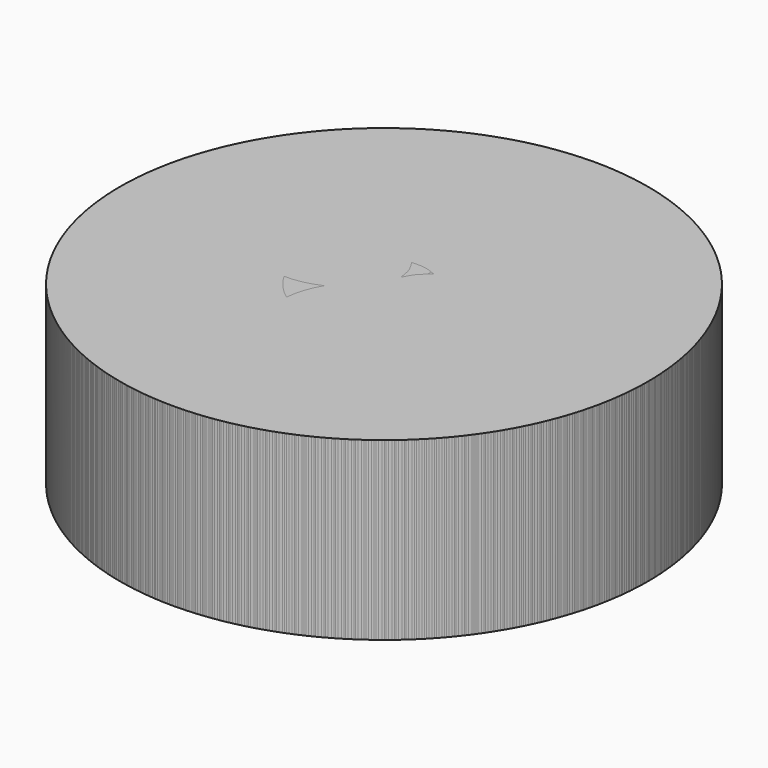
from build123d import *

# Parameters (mm, degrees)
F1_R      = 90
F2_DEPTH  = 60
F3_R      = 85
F3_R_2    = 75
F4_DEPTH  = 4
F5_R      = 75
F7_DEPTH  = 50
F8_DEPTH  = 10
F9_COUNT  = 9
F11_DEPTH = 10
F12_COUNT = 12


with BuildPart() as f2:
    # F1 (on Top) → F2 (new body)
    with BuildSketch(Plane.XY):
        Circle(F1_R)
    extrude(amount=-F2_DEPTH)

    # F3 (on face) → F4 (cut)
    with BuildSketch(Plane(origin=(0, 0, -60), x_dir=(1, 0, 0), z_dir=(0, 0, -1))):
        Circle(F3_R)
        Circle(F3_R_2, mode=Mode.SUBTRACT)
    extrude(amount=-F4_DEPTH, mode=Mode.SUBTRACT)

    # F5 (on face) → F7 (cut)
    with BuildSketch(Plane(origin=(0, 0, -60), x_dir=(1, 0, 0), z_dir=(0, 0, -1))):
        Circle(F5_R)
    extrude(amount=-F7_DEPTH, mode=Mode.SUBTRACT)

    # F0 (on Top) → F8 (cut, through all)
    with BuildSketch(Plane.XY):
        with BuildLine():
            add(Edge.make_bspline(
                [(-4.5, -13.7942286341), (-1.4705771366, -10.347114317), (-1.4705771366, -10.347114317), (0, -6)],
                knots=[0, 0, 0, 0, 9, 9, 9, 9], degree=3))
            add(Edge.make_bspline(
                [(-4.5, -13.7942286341), (0, -14.6942286341), (0, -14.6942286341), (4.5, -13.7942286341)],
                knots=[0, 0, 0, 0, 9, 9, 9, 9], degree=3))
            add(Edge.make_bspline(
                [(0, -6), (1.4705771366, -10.347114317), (1.4705771366, -10.347114317), (4.5, -13.7942286341)],
                knots=[0, 0, 0, 0, 9, 9, 9, 9], degree=3))
        make_face()
    extrude(amount=-F8_DEPTH, mode=Mode.SUBTRACT)


with BuildPart() as f9_1:
    # F9: instance of F2
    add(f2.part.rotate(Axis((0, 0, -60), (0, 0, -1)), 1 * 360 / F9_COUNT))


with BuildPart() as f9_2:
    # F9: instance of F2
    add(f2.part.rotate(Axis((0, 0, -60), (0, 0, -1)), 2 * 360 / F9_COUNT))


with BuildPart() as f9_3:
    # F9: instance of F2
    add(f2.part.rotate(Axis((0, 0, -60), (0, 0, -1)), 3 * 360 / F9_COUNT))


with BuildPart() as f9_4:
    # F9: instance of F2
    add(f2.part.rotate(Axis((0, 0, -60), (0, 0, -1)), 4 * 360 / F9_COUNT))


with BuildPart() as f9_5:
    # F9: instance of F2
    add(f2.part.rotate(Axis((0, 0, -60), (0, 0, -1)), 5 * 360 / F9_COUNT))


with BuildPart() as f9_6:
    # F9: instance of F2
    add(f2.part.rotate(Axis((0, 0, -60), (0, 0, -1)), 6 * 360 / F9_COUNT))


with BuildPart() as f9_7:
    # F9: instance of F2
    add(f2.part.rotate(Axis((0, 0, -60), (0, 0, -1)), 7 * 360 / F9_COUNT))


with BuildPart() as f9_8:
    # F9: instance of F2
    add(f2.part.rotate(Axis((0, 0, -60), (0, 0, -1)), 8 * 360 / F9_COUNT))


with BuildPart() as f11_tool:
    # F10 (on face) → F11 (new body, through all)
    with BuildSketch(Plane.XY):
        with BuildLine():
            ThreePointArc((-4.9412984546, -15.1469779182), (-8.9537537737, -19.6587371709), (-13.868495, -23.1660278519))
            ThreePointArc((-13.868495, -23.1660278519), (-8.3737215587, -25.6686732664), (-2.4601957705, -26.887681878))
            ThreePointArc((-2.4601957705, -26.887681878), (-4.3612662396, -21.1569140137), (-4.9412984546, -15.1469779182))
        make_face()
    extrude(amount=-F11_DEPTH)


with BuildPart() as f2_1:
    add(f2.part)

    # F11: cut by f11_tool
    add(f11_tool.part, mode=Mode.SUBTRACT)


with BuildPart() as f9_1_1:
    add(f9_1.part)

    # F11: cut by f11_tool
    add(f11_tool.part, mode=Mode.SUBTRACT)


with BuildPart() as f9_2_1:
    add(f9_2.part)

    # F11: cut by f11_tool
    add(f11_tool.part, mode=Mode.SUBTRACT)


with BuildPart() as f9_3_1:
    add(f9_3.part)

    # F11: cut by f11_tool
    add(f11_tool.part, mode=Mode.SUBTRACT)


with BuildPart() as f9_4_1:
    add(f9_4.part)

    # F11: cut by f11_tool
    add(f11_tool.part, mode=Mode.SUBTRACT)


with BuildPart() as f9_5_1:
    add(f9_5.part)

    # F11: cut by f11_tool
    add(f11_tool.part, mode=Mode.SUBTRACT)


with BuildPart() as f9_6_1:
    add(f9_6.part)

    # F11: cut by f11_tool
    add(f11_tool.part, mode=Mode.SUBTRACT)


with BuildPart() as f9_7_1:
    add(f9_7.part)

    # F11: cut by f11_tool
    add(f11_tool.part, mode=Mode.SUBTRACT)


with BuildPart() as f9_8_1:
    add(f9_8.part)

    # F11: cut by f11_tool
    add(f11_tool.part, mode=Mode.SUBTRACT)


with BuildPart() as f12_1:
    # F12: instance of F9_4
    add(f9_4_1.part.rotate(Axis((0, 0, 0), (0, 0, 1)), 1 * 360 / F12_COUNT))


with BuildPart() as f12_2:
    # F12: instance of F9_4
    add(f9_4_1.part.rotate(Axis((0, 0, 0), (0, 0, 1)), 2 * 360 / F12_COUNT))


with BuildPart() as f12_3:
    # F12: instance of F9_4
    add(f9_4_1.part.rotate(Axis((0, 0, 0), (0, 0, 1)), 3 * 360 / F12_COUNT))


with BuildPart() as f12_4:
    # F12: instance of F9_4
    add(f9_4_1.part.rotate(Axis((0, 0, 0), (0, 0, 1)), 4 * 360 / F12_COUNT))


with BuildPart() as f12_5:
    # F12: instance of F9_4
    add(f9_4_1.part.rotate(Axis((0, 0, 0), (0, 0, 1)), 5 * 360 / F12_COUNT))


with BuildPart() as f12_6:
    # F12: instance of F9_4
    add(f9_4_1.part.rotate(Axis((0, 0, 0), (0, 0, 1)), 6 * 360 / F12_COUNT))


with BuildPart() as f12_7:
    # F12: instance of F9_4
    add(f9_4_1.part.rotate(Axis((0, 0, 0), (0, 0, 1)), 7 * 360 / F12_COUNT))


with BuildPart() as f12_8:
    # F12: instance of F9_4
    add(f9_4_1.part.rotate(Axis((0, 0, 0), (0, 0, 1)), 8 * 360 / F12_COUNT))


with BuildPart() as f12_9:
    # F12: instance of F9_4
    add(f9_4_1.part.rotate(Axis((0, 0, 0), (0, 0, 1)), 9 * 360 / F12_COUNT))


with BuildPart() as f12_10:
    # F12: instance of F9_4
    add(f9_4_1.part.rotate(Axis((0, 0, 0), (0, 0, 1)), 10 * 360 / F12_COUNT))


with BuildPart() as f12_11:
    # F12: instance of F9_4
    add(f9_4_1.part.rotate(Axis((0, 0, 0), (0, 0, 1)), 11 * 360 / F12_COUNT))


solid = Compound([f2_1.part, f9_1_1.part, f9_2_1.part, f9_3_1.part, f9_4_1.part, f9_5_1.part, f9_6_1.part, f9_7_1.part, f9_8_1.part, f12_1.part, f12_2.part, f12_3.part, f12_4.part, f12_5.part, f12_6.part, f12_7.part, f12_8.part, f12_9.part, f12_10.part, f12_11.part])
